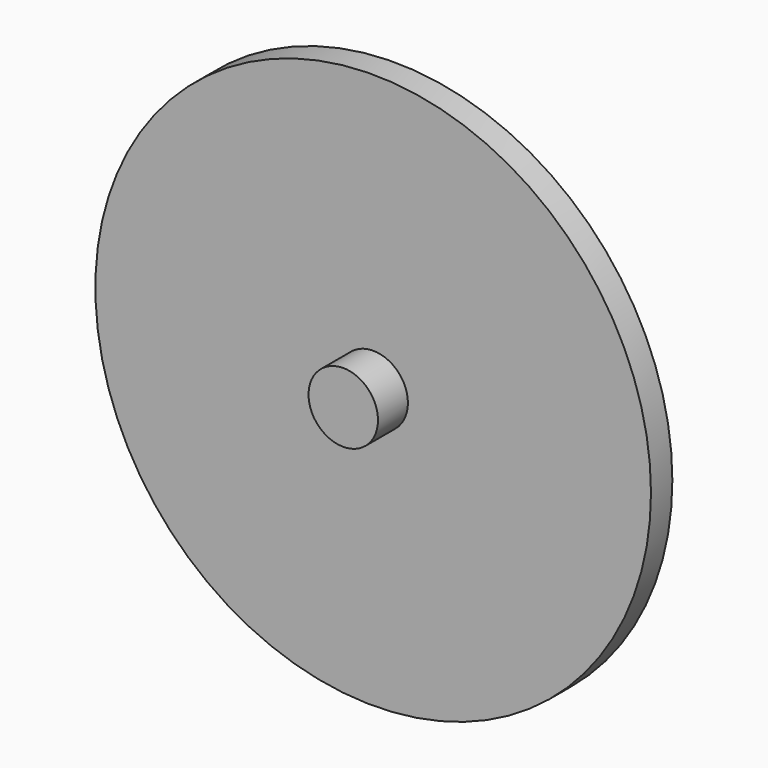
from build123d import *

# Parameters (mm, degrees)
F0_R     = 66.04
F1_DEPTH = 6.35
F2_R     = 8.255
F3_DEPTH = 15.24


# Not quite as in the source:
# - a feature names something its author has since deleted; it is built from what else it names


with BuildPart() as f1:
    # F0 (on Front) → F1 (new body)
    with BuildSketch(Plane.XZ):
        Circle(F0_R)
    extrude(amount=F1_DEPTH)

    # F2 (on Front) → F3 (join)
    with BuildSketch(Plane.XZ):
        Circle(F2_R)
    extrude(amount=F3_DEPTH)


solid = f1.part
